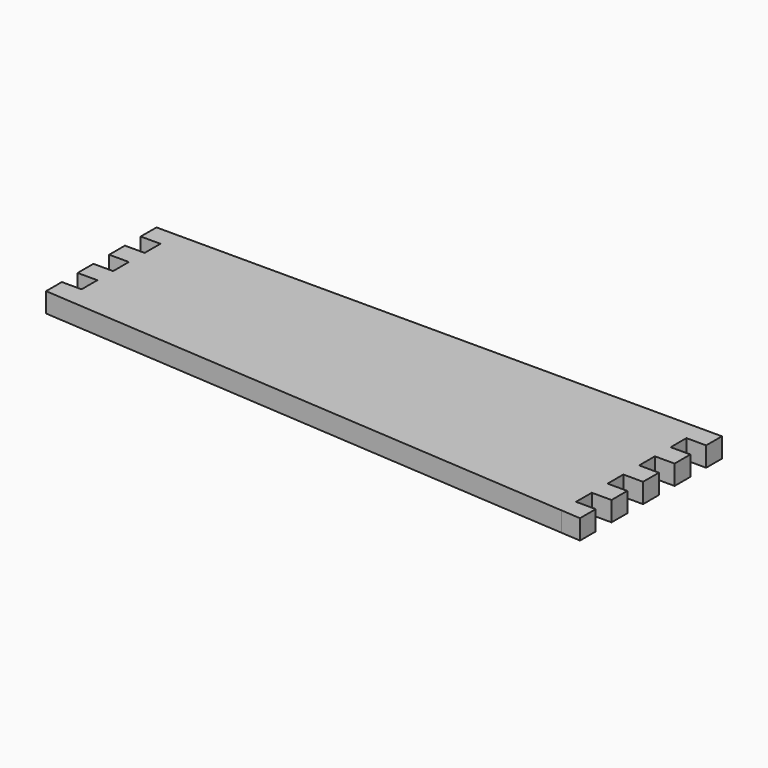
from build123d import *

# Parameters (mm, degrees)
F0_W     = 10
F0_H     = 10
F1_DEPTH = 10


# Not quite as in the source:
# - a feature names something its author has since deleted; it is built from what else it names


with BuildPart() as f1:
    # F0 (on Top) → F1 (new body)
    with BuildSketch(Plane.XY):
        Polygon((131.1653250098, 36.9413525529), (-135.6346749902, 36.9413525529), (-135.6346749902, 26.9413525529), (-135.6346749902, 16.9413525529), (-135.6346749902, 6.9413525529), (-135.6346749902, -3.0586474471), (-135.6346749902, -13.0586474471), (-135.6346749902, -23.0586474471), (-135.6346749902, -33.0586474471), (131.1653250098, -33.0586474471), (131.1653250098, -23.0586474471), (131.1653250098, -13.0586474471), (131.1653250098, -3.0586474471), (131.1653250098, 6.9413525529), (131.1653250098, 16.9413525529), (131.1653250098, 26.9413525529), align=None)
        with Locations((-140.6346749902, 31.9413525529)):
            Rectangle(F0_W, F0_H)
        with Locations((-140.6346749902, 11.9413525529)):
            Rectangle(F0_W, F0_H)
        with Locations((-140.6346749902, -8.0586474471)):
            Rectangle(F0_W, F0_H)
        with Locations((-140.6346749902, -28.0586474471)):
            Rectangle(F0_W, F0_H)
        with Locations((136.1653250098, 31.9413525529)):
            Rectangle(F0_W, F0_H)
        with Locations((136.1653250098, 11.9413525529)):
            Rectangle(F0_W, F0_H)
        with Locations((136.1653250098, -8.0586474471)):
            Rectangle(F0_W, F0_H)
        with Locations((136.1653250098, -28.0586474471)):
            Rectangle(F0_W, F0_H)
        Polygon((-135.6346749902, -33.0586474471), (-145.6346749902, -33.0586474471), (131.1653250098, -52.3612973773), (131.1653250098, -43.0586474471), (131.1653250098, -33.0586474471), align=None)
        Polygon((131.1653250098, -43.0586474471), (131.1653250098, -52.3612973773), (141.1653250098, -53.0586474471), (141.1653250098, -43.0586474471), align=None)
    extrude(amount=F1_DEPTH)


solid = f1.part
